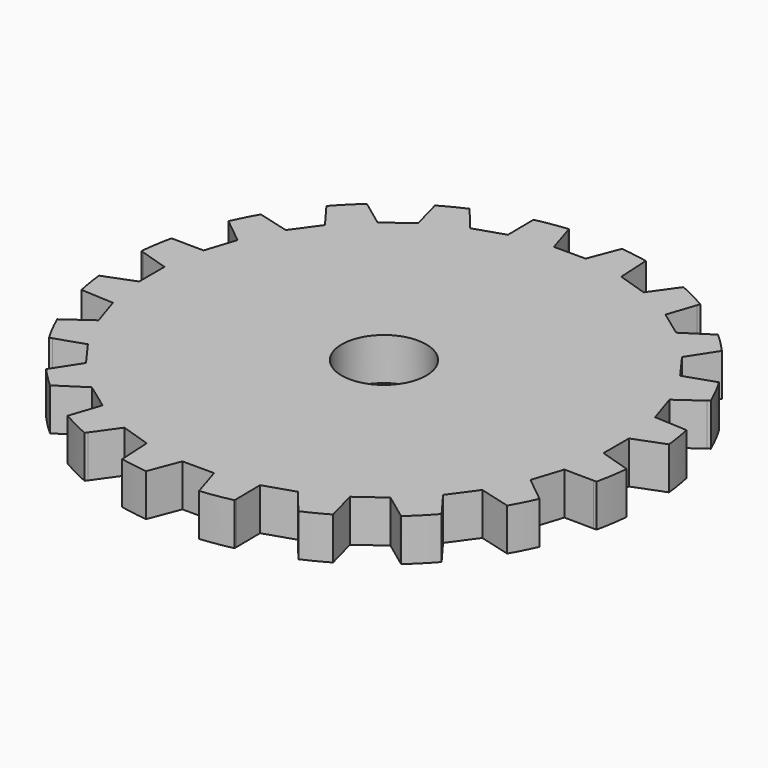
from build123d import *

# Parameters (mm, degrees)
F0_R            = 12.5
F1_DEPTH        = 2
F4_R            = 2
F5_DEPTH        = 2.001
F6_DEPTH        = 25
F6_COPIES_COUNT = 10


# Not quite as in the source:
# - a pattern or mirror of a feature is missing from the dataset's text; its kind, count and spacing are read off the source's solid


with BuildPart() as f1:
    # F0 (on Top) → F1 (new body)
    with BuildSketch(Plane.XY):
        Circle(F0_R)
    extrude(amount=-F1_DEPTH)

    # F4 (on Top) → F5 (cut, through all)
    with BuildSketch(Plane.XY):
        Circle(F4_R)
    extrude(amount=-F5_DEPTH, mode=Mode.SUBTRACT)

    # F2 (on Top) → F6 (cut)
    with BuildSketch(Plane.XY):
        Polygon((-4.1068853747, 10.2126425235), (-2.6803006002, 10.6761680151), (-2.6946043422, 12.0732165994), (-2.6961970684, 12.2287784087), (-1.955430813, 12.3461042574), (-1.2146645576, 12.4634301062), (-1.1681080875, 12.3149898543), (-0.75, 10.9818975953), (0.75, 10.9818975953), (1.3061428446, 12.431572341), (-2.4499027058, 15.1036279276), (-5.0837827838, 11.4195075466), align=None)
    f6 = extrude(amount=-F6_DEPTH, mode=Mode.SUBTRACT)

    # F6_copies: F6 ×10 about axis
    f6_copies_axis = Axis((0, 0, 0), (0, 0, 1))
    for i in range(1, F6_COPIES_COUNT):
        add(f6.rotate(f6_copies_axis, i * 360 / F6_COPIES_COUNT), mode=Mode.SUBTRACT)


solid = f1.part
